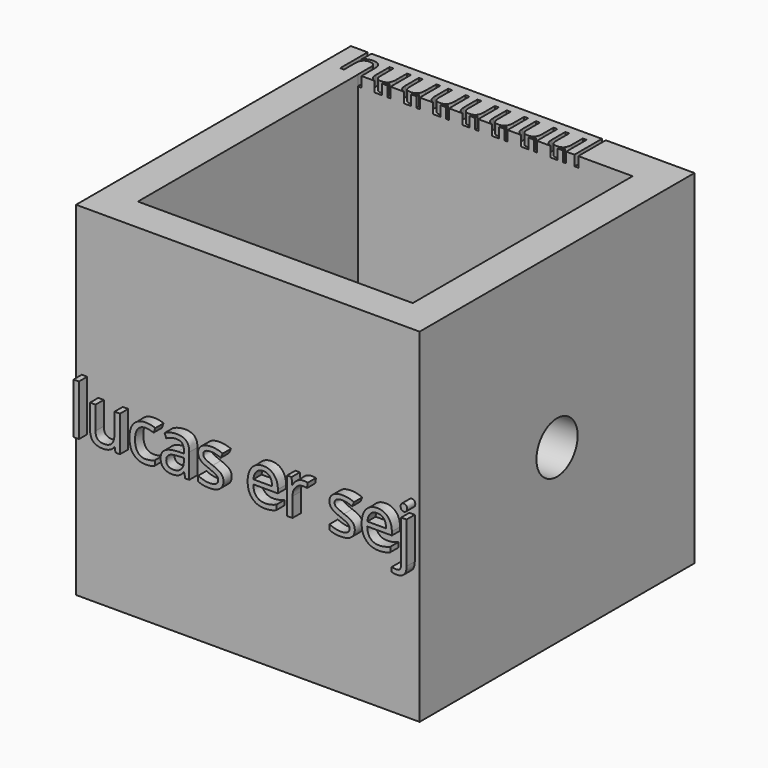
from build123d import *

# Parameters (mm, degrees)
F0_W         = 100
F0_H         = 100
F1_DEPTH     = 100
F2_T         = -10
F3_R         = 7.5
F4_DEPTH     = 100
F5_TEXT_SIZE = 19.4446132345
F6_DEPTH     = 3
F7_TEXT_SIZE = 30.3066177341
F8_DEPTH     = 3
F9_TEXT_SIZE = 13.8888888889
F10_DEPTH    = 3


# Not quite as in the source:
# - Text() gives the source's letters only with a copy of the font that has no kerning and outlines rounded to 1/6400 em; it was checked with that copy


with BuildPart() as f1:
    # F0 (on Top) → F1 (new body)
    with BuildSketch(Plane.XY):
        with Locations((50, 50)):
            Rectangle(F0_W, F0_H)
    extrude(amount=F1_DEPTH)

    # F2
    f2_openings = [f1.faces().sort_by_distance(p)[0] for p in [
        (50, 50, 100),
    ]]
    offset(amount=F2_T, openings=f2_openings)

    # F3 (on face) → F4 (cut)
    with BuildSketch(Plane(origin=(0, 0, 0), x_dir=(0, -1, 0), z_dir=(-1, 0, 0))):
        with Locations((-50, 50)):
            Circle(F3_R)
    extrude(amount=-F4_DEPTH, mode=Mode.SUBTRACT)

    # F5 (on face) → F6 (join)
    with BuildSketch(Plane.XZ):
        with Locations((0, 42.2155049857)):
            Text('lucas er sej', F5_TEXT_SIZE, font='Open Sans', text_align=(TextAlign.LEFT, TextAlign.BOTTOM))
    extrude(amount=F6_DEPTH)

    # F7 (on face) → F8 (join)
    with BuildSketch(Plane(origin=(0, 10, 0), x_dir=(-1, 0, 0), z_dir=(0, 1, 0))):
        with Locations((-90, 32.8137453137)):
            Text('hulen', F7_TEXT_SIZE, font='Open Sans', text_align=(TextAlign.LEFT, TextAlign.BOTTOM))
    extrude(amount=F8_DEPTH)

    # F9 (on face) → F10 (cut)
    with BuildSketch(Plane.XY.offset(100)):
        with Locations((3.6743865824, 90)):
            Text('huuuuuuul', F9_TEXT_SIZE, font='Open Sans', text_align=(TextAlign.LEFT, TextAlign.BOTTOM))
    extrude(amount=-F10_DEPTH, mode=Mode.SUBTRACT)


solid = f1.part
